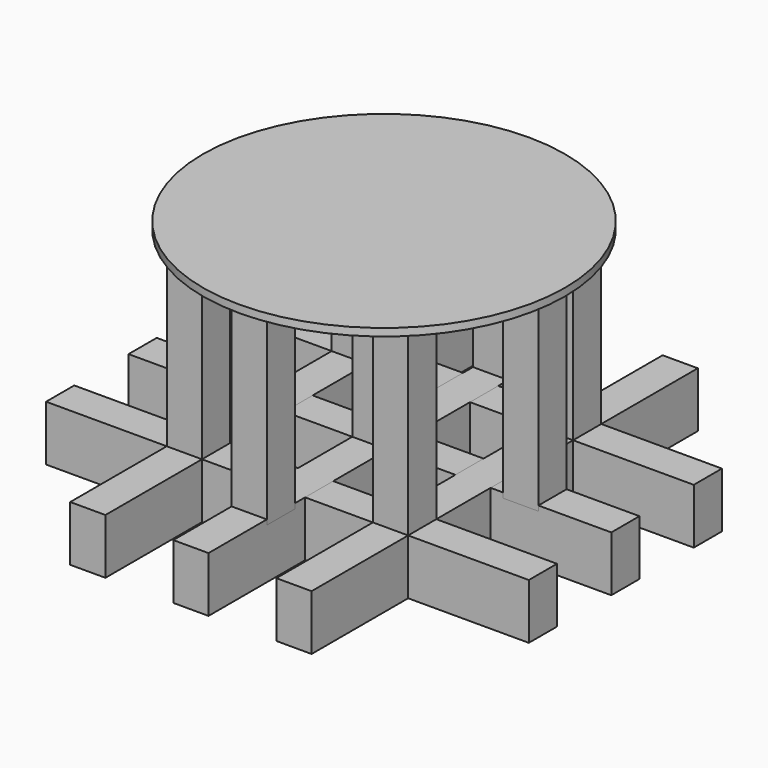
from build123d import *

# Parameters (mm, degrees)
F0_W          = 88.9
F0_H          = 304.8
F0_H_2        = 88.9
F0_H_3        = 171.45
F1_DEPTH      = 139.7
F0_W_2        = 304.8
F0_W_3        = 171.45
F2_DEPTH      = 139.7
F3_W          = 88.9
F3_H          = 69.85
F4_DEPTH      = 914.401
F5_W          = 88.9
F5_H          = 69.85
F6_DEPTH      = 914.401
F7_W          = 88.9
F7_H          = 88.9
F8_DEPTH      = 457.2
F8_DEPTH_BACK = 12.7
F10_R         = 457.2
F10_W         = 88.9
F10_H         = 88.9
F11_DEPTH     = 19.05


# Not quite as in the source:
# - a feature names something its author has since deleted; it is built from what else it names


with BuildPart() as f1:
    # F0 (on Top) → F1 (new body)
    with BuildSketch(Plane.XY):
        with Locations((-260.35, 457.2)):
            Rectangle(F0_W, F0_H)
        with Locations((-260.35, 260.35)):
            Rectangle(F0_W, F0_H_2)
        with Locations((-260.35, 130.175)):
            Rectangle(F0_W, F0_H_3)
        with Locations((-260.35, 0)):
            Rectangle(F0_W, F0_H_2)
        with Locations((-260.35, -130.175)):
            Rectangle(F0_W, F0_H_3)
        with Locations((-260.35, -260.35)):
            Rectangle(F0_W, F0_H_2)
        with Locations((-260.35, -457.2)):
            Rectangle(F0_W, F0_H)
    extrude(amount=F1_DEPTH)


with BuildPart() as f1b:
    # F0 (on Top) → F1, piece 2 (new body)
    with BuildSketch(Plane.XY):
        with Locations((0, -457.2)):
            Rectangle(F0_W, F0_H)
        with Locations((0, -260.35)):
            Rectangle(F0_W, F0_H_2)
        with Locations((0, -130.175)):
            Rectangle(F0_W, F0_H_3)
        Rectangle(F0_W, F0_H_2)
        with Locations((0, 130.175)):
            Rectangle(F0_W, F0_H_3)
        with Locations((0, 260.35)):
            Rectangle(F0_W, F0_H_2)
        with Locations((0, 457.2)):
            Rectangle(F0_W, F0_H)
    extrude(amount=F1_DEPTH)


with BuildPart() as f1c:
    # F0 (on Top) → F1, piece 3 (new body)
    with BuildSketch(Plane.XY):
        with Locations((260.35, 457.2)):
            Rectangle(F0_W, F0_H)
        with Locations((260.35, 260.35)):
            Rectangle(F0_W, F0_H_2)
        with Locations((260.35, 130.175)):
            Rectangle(F0_W, F0_H_3)
        with Locations((260.35, 0)):
            Rectangle(F0_W, F0_H_2)
        with Locations((260.35, -130.175)):
            Rectangle(F0_W, F0_H_3)
        with Locations((260.35, -260.35)):
            Rectangle(F0_W, F0_H_2)
        with Locations((260.35, -457.2)):
            Rectangle(F0_W, F0_H)
    extrude(amount=F1_DEPTH)


with BuildPart() as f2:
    # F0 (on Top) → F2 (new body)
    with BuildSketch(Plane.XY):
        with Locations((-457.2, 260.35)):
            Rectangle(F0_W_2, F0_H_2)
        with Locations((-260.35, 260.35)):
            Rectangle(F0_W, F0_H_2)
        with Locations((-130.175, 260.35)):
            Rectangle(F0_W_3, F0_H_2)
        with Locations((0, 260.35)):
            Rectangle(F0_W, F0_H_2)
        with Locations((130.175, 260.35)):
            Rectangle(F0_W_3, F0_H_2)
        with Locations((260.35, 260.35)):
            Rectangle(F0_W, F0_H_2)
        with Locations((457.2, 260.35)):
            Rectangle(F0_W_2, F0_H_2)
    extrude(amount=F2_DEPTH)


with BuildPart() as f2b:
    # F0 (on Top) → F2, piece 2 (new body)
    with BuildSketch(Plane.XY):
        with Locations((457.2, 0)):
            Rectangle(F0_W_2, F0_H_2)
        with Locations((260.35, 0)):
            Rectangle(F0_W, F0_H_2)
        with Locations((130.175, 0)):
            Rectangle(F0_W_3, F0_H_2)
        Rectangle(F0_W, F0_H_2)
        with Locations((-130.175, 0)):
            Rectangle(F0_W_3, F0_H_2)
        with Locations((-260.35, 0)):
            Rectangle(F0_W, F0_H_2)
        with Locations((-457.2, 0)):
            Rectangle(F0_W_2, F0_H_2)
    extrude(amount=F2_DEPTH)


with BuildPart() as f2c:
    # F0 (on Top) → F2, piece 3 (new body)
    with BuildSketch(Plane.XY):
        with Locations((-457.2, -260.35)):
            Rectangle(F0_W_2, F0_H_2)
        with Locations((-260.35, -260.35)):
            Rectangle(F0_W, F0_H_2)
        with Locations((-130.175, -260.35)):
            Rectangle(F0_W_3, F0_H_2)
        with Locations((0, -260.35)):
            Rectangle(F0_W, F0_H_2)
        with Locations((130.175, -260.35)):
            Rectangle(F0_W_3, F0_H_2)
        with Locations((260.35, -260.35)):
            Rectangle(F0_W, F0_H_2)
        with Locations((457.2, -260.35)):
            Rectangle(F0_W_2, F0_H_2)
    extrude(amount=F2_DEPTH)


with BuildPart() as f4_tool:
    # F3 (on face) → F4 (new body, through all)
    with BuildSketch(Plane.XZ.offset(304.8)):
        with Locations((-260.35, 104.775)):
            Rectangle(F3_W, F3_H)
        with Locations((0, 104.775)):
            Rectangle(F3_W, F3_H)
        with Locations((260.35, 104.775)):
            Rectangle(F3_W, F3_H)
    extrude(amount=-F4_DEPTH)


with BuildPart() as f2_1:
    add(f2.part)

    # F4: cut by f4_tool
    add(f4_tool.part, mode=Mode.SUBTRACT)


with BuildPart() as f2b_1:
    add(f2b.part)

    # F4: cut by f4_tool
    add(f4_tool.part, mode=Mode.SUBTRACT)


with BuildPart() as f2c_1:
    add(f2c.part)

    # F4: cut by f4_tool
    add(f4_tool.part, mode=Mode.SUBTRACT)


with BuildPart() as f6_tool:
    # F5 (on face) → F6 (new body, through all)
    with BuildSketch(Plane.YZ.offset(304.8)):
        with Locations((-260.35, 34.925)):
            Rectangle(F5_W, F5_H)
        with Locations((0, 34.925)):
            Rectangle(F5_W, F5_H)
        with Locations((260.35, 34.925)):
            Rectangle(F5_W, F5_H)
    extrude(amount=-F6_DEPTH)


with BuildPart() as f1_1:
    add(f1.part)

    # F6: cut by f6_tool
    add(f6_tool.part, mode=Mode.SUBTRACT)


with BuildPart() as f1b_1:
    add(f1b.part)

    # F6: cut by f6_tool
    add(f6_tool.part, mode=Mode.SUBTRACT)


with BuildPart() as f1c_1:
    add(f1c.part)

    # F6: cut by f6_tool
    add(f6_tool.part, mode=Mode.SUBTRACT)


with BuildPart() as f8:
    # F7 (on face) → F8 (new body, two sides)
    with BuildSketch(Plane.XY.offset(139.7)) as f8_sk:
        with Locations((-260.35, 260.35)):
            Rectangle(F7_W, F7_H)
    extrude(amount=F8_DEPTH)
    extrude(f8_sk.sketch, amount=-F8_DEPTH_BACK)


with BuildPart() as f8b:
    # F7 (on face) → F8, piece 2 (new body, two sides)
    with BuildSketch(Plane.XY.offset(139.7)) as f8_2_sk:
        with Locations((260.35, 260.35)):
            Rectangle(F7_W, F7_H)
    extrude(amount=F8_DEPTH)
    extrude(f8_2_sk.sketch, amount=-F8_DEPTH_BACK)


with BuildPart() as f8c:
    # F7 (on face) → F8, piece 3 (new body, two sides)
    with BuildSketch(Plane.XY.offset(139.7)) as f8_3_sk:
        Rectangle(F7_W, F7_H)
    extrude(amount=F8_DEPTH)
    extrude(f8_3_sk.sketch, amount=-F8_DEPTH_BACK)


with BuildPart() as f8d:
    # F7 (on face) → F8, piece 4 (new body, two sides)
    with BuildSketch(Plane.XY.offset(139.7)) as f8_4_sk:
        with Locations((0, 381)):
            Rectangle(F7_W, F7_H)
    extrude(amount=F8_DEPTH)
    extrude(f8_4_sk.sketch, amount=-F8_DEPTH_BACK)


with BuildPart() as f8e:
    # F7 (on face) → F8, piece 5 (new body, two sides)
    with BuildSketch(Plane.XY.offset(139.7)) as f8_5_sk:
        with Locations((0, -381)):
            Rectangle(F7_W, F7_H)
    extrude(amount=F8_DEPTH)
    extrude(f8_5_sk.sketch, amount=-F8_DEPTH_BACK)


with BuildPart() as f8f:
    # F7 (on face) → F8, piece 6 (new body, two sides)
    with BuildSketch(Plane.XY.offset(139.7)) as f8_6_sk:
        with Locations((-260.35, -260.35)):
            Rectangle(F7_W, F7_H)
    extrude(amount=F8_DEPTH)
    extrude(f8_6_sk.sketch, amount=-F8_DEPTH_BACK)


with BuildPart() as f8g:
    # F7 (on face) → F8, piece 7 (new body, two sides)
    with BuildSketch(Plane.XY.offset(139.7)) as f8_7_sk:
        with Locations((260.35, -260.35)):
            Rectangle(F7_W, F7_H)
    extrude(amount=F8_DEPTH)
    extrude(f8_7_sk.sketch, amount=-F8_DEPTH_BACK)


with BuildPart() as f8h:
    # F7 (on face) → F8, piece 8 (new body, two sides)
    with BuildSketch(Plane.XY.offset(139.7)) as f8_8_sk:
        with Locations((381, 0)):
            Rectangle(F7_W, F7_H)
    extrude(amount=F8_DEPTH)
    extrude(f8_8_sk.sketch, amount=-F8_DEPTH_BACK)


with BuildPart() as f8i:
    # F7 (on face) → F8, piece 9 (new body, two sides)
    with BuildSketch(Plane.XY.offset(139.7)) as f8_9_sk:
        with Locations((-381, 0)):
            Rectangle(F7_W, F7_H)
    extrude(amount=F8_DEPTH)
    extrude(f8_9_sk.sketch, amount=-F8_DEPTH_BACK)


with BuildPart() as f1_2:
    add(f1_1.part)

    # F9: cut F8i, F8, F8d, F8b, F8h, F8c, F8g, F8e, F8f
    add(f8i.part, mode=Mode.SUBTRACT)
    add(f8.part, mode=Mode.SUBTRACT)
    add(f8d.part, mode=Mode.SUBTRACT)
    add(f8b.part, mode=Mode.SUBTRACT)
    add(f8h.part, mode=Mode.SUBTRACT)
    add(f8c.part, mode=Mode.SUBTRACT)
    add(f8g.part, mode=Mode.SUBTRACT)
    add(f8e.part, mode=Mode.SUBTRACT)
    add(f8f.part, mode=Mode.SUBTRACT)


with BuildPart() as f2b_2:
    add(f2b_1.part)

    # F9: cut F8i, F8, F8d, F8b, F8h, F8c, F8g, F8e, F8f
    add(f8i.part, mode=Mode.SUBTRACT)
    add(f8.part, mode=Mode.SUBTRACT)
    add(f8d.part, mode=Mode.SUBTRACT)
    add(f8b.part, mode=Mode.SUBTRACT)
    add(f8h.part, mode=Mode.SUBTRACT)
    add(f8c.part, mode=Mode.SUBTRACT)
    add(f8g.part, mode=Mode.SUBTRACT)
    add(f8e.part, mode=Mode.SUBTRACT)
    add(f8f.part, mode=Mode.SUBTRACT)


with BuildPart() as f2_2:
    add(f2_1.part)

    # F9: cut F8i, F8, F8d, F8b, F8h, F8c, F8g, F8e, F8f
    add(f8i.part, mode=Mode.SUBTRACT)
    add(f8.part, mode=Mode.SUBTRACT)
    add(f8d.part, mode=Mode.SUBTRACT)
    add(f8b.part, mode=Mode.SUBTRACT)
    add(f8h.part, mode=Mode.SUBTRACT)
    add(f8c.part, mode=Mode.SUBTRACT)
    add(f8g.part, mode=Mode.SUBTRACT)
    add(f8e.part, mode=Mode.SUBTRACT)
    add(f8f.part, mode=Mode.SUBTRACT)


with BuildPart() as f1c_2:
    add(f1c_1.part)

    # F9: cut F8i, F8, F8d, F8b, F8h, F8c, F8g, F8e, F8f
    add(f8i.part, mode=Mode.SUBTRACT)
    add(f8.part, mode=Mode.SUBTRACT)
    add(f8d.part, mode=Mode.SUBTRACT)
    add(f8b.part, mode=Mode.SUBTRACT)
    add(f8h.part, mode=Mode.SUBTRACT)
    add(f8c.part, mode=Mode.SUBTRACT)
    add(f8g.part, mode=Mode.SUBTRACT)
    add(f8e.part, mode=Mode.SUBTRACT)
    add(f8f.part, mode=Mode.SUBTRACT)


with BuildPart() as f1b_2:
    add(f1b_1.part)

    # F9: cut F8i, F8, F8d, F8b, F8h, F8c, F8g, F8e, F8f
    add(f8i.part, mode=Mode.SUBTRACT)
    add(f8.part, mode=Mode.SUBTRACT)
    add(f8d.part, mode=Mode.SUBTRACT)
    add(f8b.part, mode=Mode.SUBTRACT)
    add(f8h.part, mode=Mode.SUBTRACT)
    add(f8c.part, mode=Mode.SUBTRACT)
    add(f8g.part, mode=Mode.SUBTRACT)
    add(f8e.part, mode=Mode.SUBTRACT)
    add(f8f.part, mode=Mode.SUBTRACT)


with BuildPart() as f2c_2:
    add(f2c_1.part)

    # F9: cut F8i, F8, F8d, F8b, F8h, F8c, F8g, F8e, F8f
    add(f8i.part, mode=Mode.SUBTRACT)
    add(f8.part, mode=Mode.SUBTRACT)
    add(f8d.part, mode=Mode.SUBTRACT)
    add(f8b.part, mode=Mode.SUBTRACT)
    add(f8h.part, mode=Mode.SUBTRACT)
    add(f8c.part, mode=Mode.SUBTRACT)
    add(f8g.part, mode=Mode.SUBTRACT)
    add(f8e.part, mode=Mode.SUBTRACT)
    add(f8f.part, mode=Mode.SUBTRACT)


with BuildPart() as f11:
    # F10 (on face) → F11 (new body)
    with BuildSketch(Plane.XY.offset(596.9)):
        Circle(F10_R)
        Rectangle(F10_W, F10_H, mode=Mode.SUBTRACT)
        Rectangle(F10_W, F10_H)
    extrude(amount=F11_DEPTH)


solid = Compound([f8.part, f8b.part, f8c.part, f8d.part, f8e.part, f8f.part, f8g.part, f8h.part, f8i.part, f1_2.part, f2b_2.part, f2_2.part, f1c_2.part, f1b_2.part, f2c_2.part, f11.part])
